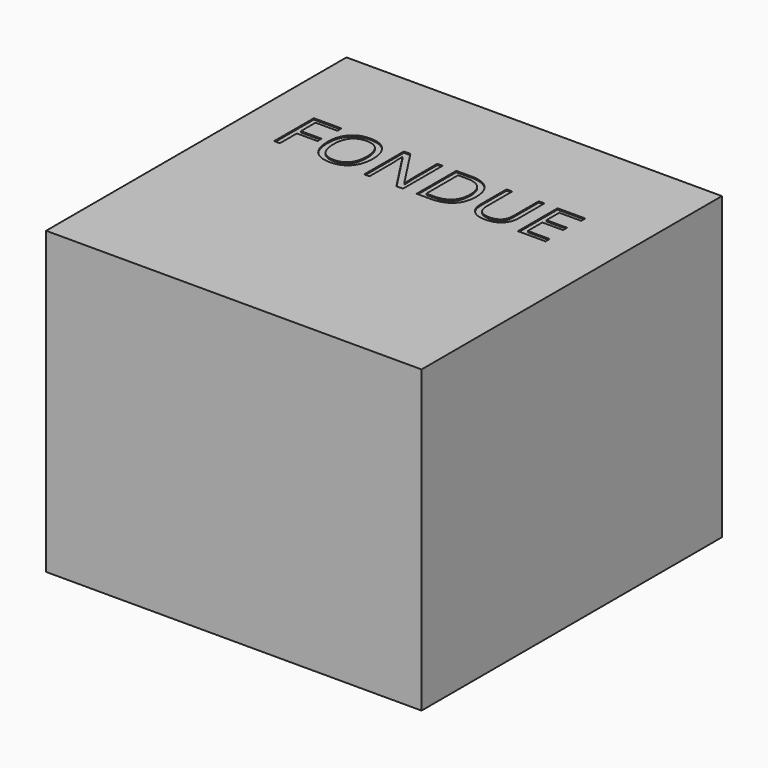
from build123d import *

# Parameters (mm, degrees)
F0_W         = 300
F0_H         = 300
F1_DEPTH     = 240
F2_TEXT_SIZE = 55.5555555556
F3_DEPTH     = 1


# Not quite as in the source:
# - Text() gives the source's letters only with a copy of the font that has no kerning and outlines rounded to 1/6400 em; it was checked with that copy


with BuildPart() as f1:
    # F0 (on Top) → F1 (new body)
    with BuildSketch(Plane.XY):
        Rectangle(F0_W, F0_H)
    extrude(amount=F1_DEPTH)

    # F2 (on face) → F3 (cut)
    with BuildSketch(Plane.XY.offset(240)):
        with Locations((-120, 33.4592628217)):
            Text('FONDUE', F2_TEXT_SIZE, font='Open Sans', text_align=(TextAlign.LEFT, TextAlign.BOTTOM))
    extrude(amount=-F3_DEPTH, mode=Mode.SUBTRACT)


solid = f1.part
